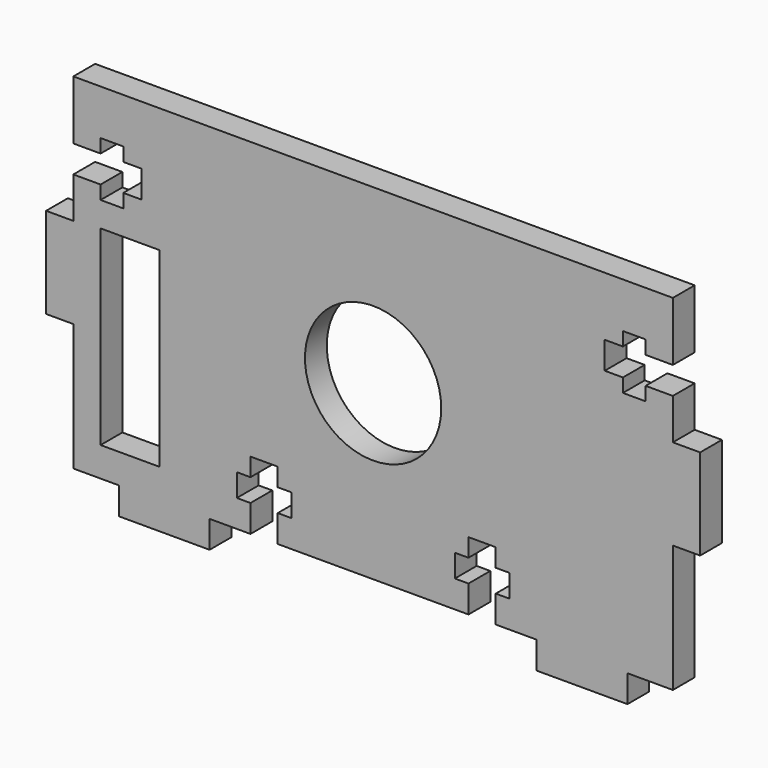
from build123d import *

# Parameters (mm, degrees)
F1_W     = 6.5
F1_H     = 21
F1_R     = 7.5
F2_DEPTH = 3
F4_DEPTH = 3


# Not quite as in the source:
# - a feature names something its author has since deleted; it is built from what else it names


with BuildPart() as f2:
    # F1 (on Front) → F2 (new body)
    with BuildSketch(Plane.XZ):
        Polygon((33, 5), (33, 19), (-33, 19), (-33, 5), (-36, 5), (-36, -5), (-33, -5), (-33, -19), (-28, -19), (-28, -22), (-18, -22), (-18, -19), (0, -19), (18, -19), (18, -22), (28, -22), (28, -19), (33, -19), (33, -5), (36, -5), (36, 5), align=None)
        with Locations((-26.75, -5.25)):
            Rectangle(F1_W, F1_H, mode=Mode.SUBTRACT)
        Circle(F1_R, mode=Mode.SUBTRACT)
    extrude(amount=F2_DEPTH)

    # F3 (on face) → F4 (cut, through all)
    with BuildSketch(Plane.XZ.offset(3)):
        Polygon((10.5, -16), (10.5, -19), (13.5, -19), (13.5, -16), (15, -16), (15, -13.5), (13.5, -13.5), (13.5, -11.5), (10.5, -11.5), (10.5, -13.5), (9, -13.5), (9, -16), align=None)
        Polygon((-13.5, -19), (-10.5, -19), (-10.5, -16), (-9, -16), (-9, -13.5), (-10.5, -13.5), (-10.5, -11.5), (-13.5, -11.5), (-13.5, -13.5), (-15, -13.5), (-15, -16), (-13.5, -16), align=None)
        Polygon((30, 9.5), (33, 9.5), (33, 12.5), (30, 12.5), (30, 14), (27.5, 14), (27.5, 12.5), (25.5, 12.5), (25.5, 9.5), (27.5, 9.5), (27.5, 8), (30, 8), align=None)
        Polygon((-33, 12.5), (-33, 9.5), (-30, 9.5), (-30, 8), (-27.5, 8), (-27.5, 9.5), (-25.5, 9.5), (-25.5, 12.5), (-27.5, 12.5), (-27.5, 14), (-30, 14), (-30, 12.5), align=None)
    extrude(amount=-F4_DEPTH, mode=Mode.SUBTRACT)


solid = f2.part
